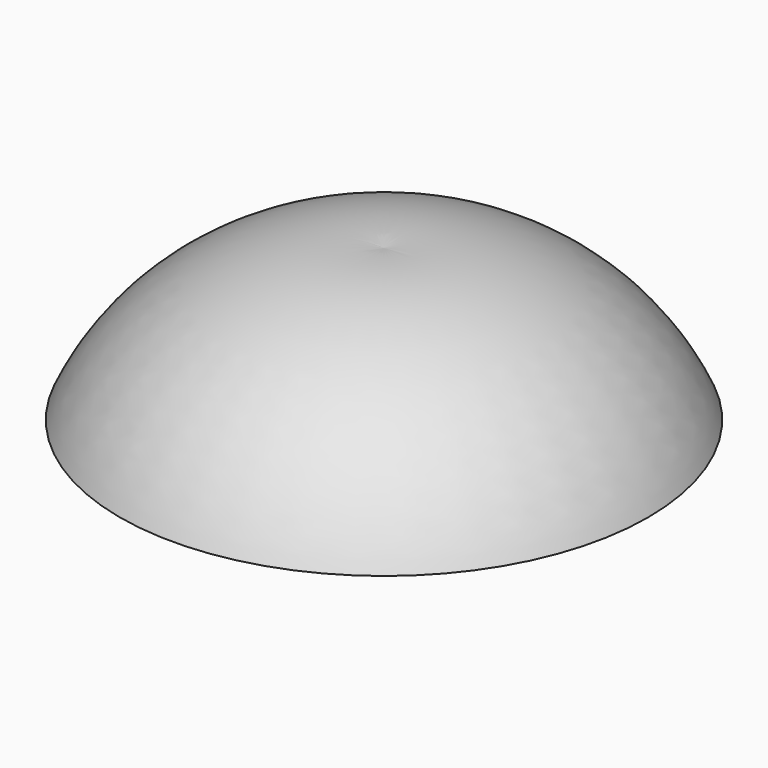
from build123d import *


with BuildPart() as f1:
    # F0 (on Front) → F1 (revolve)
    with BuildSketch(Plane.XZ):
        with BuildLine():
            ThreePointArc((34.7993297799, 20.5401515371), (12.3205620941, 45.4019329011), (-20.49517259, 52.2232763469))
            Line((-20.49517259, 52.2232763469), (-20.49517259, 40.7124921024))
            add(Edge.make_bspline(
                [(34.7993297799, 20.5401515371), (9.8439750213, 30.3270432522), (-20.49517259, 40.7124921024)],
                knots=[0.9870990838, 0.9870990838, 0.9870990838, 1.6140842113, 1.6140842113, 1.6140842113], degree=2, weights=[1, 0.951262327, 1]))
        make_face()
    revolve(axis=Axis((-20.49517259, 0, -1.4780182391), (0, 0, -1)))


solid = f1.part
